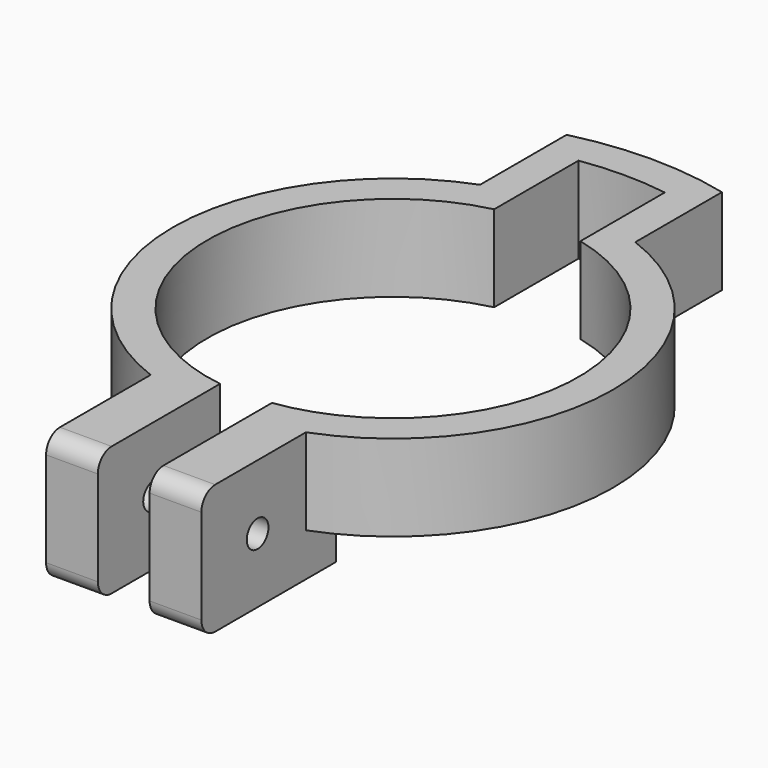
from build123d import *

# Parameters (mm, degrees)
F1_DEPTH = 5
F3_DEPTH = 7.5
F5_DEPTH = 7.5
F6_R     = 1
F7_R     = 0.7847872087
F8_DEPTH = 25


with BuildPart() as f1:
    # F0 (on Top) → F1 (new body)
    with BuildSketch(Plane.XY):
        with BuildLine():
            Line((-4.5, 18.2019916493), (-4.5, 11.9294802904))
            ThreePointArc((-4.5, 11.9294802904), (0, -12.75), (4.5, 11.9294802904))
            Line((4.5, 11.9294802904), (4.5, 18.2019916493))
            ThreePointArc((4.5, 18.2019916493), (0, 18.75), (-4.5, 18.2019916493))
        make_face()
        with BuildLine():
            ThreePointArc((2.5, 10.4552618332), (0, -10.75), (-2.5, 10.4552618332))
            Line((-2.5, 10.4552618332), (-2.5, 16.5623820751))
            ThreePointArc((-2.5, 16.5623820751), (0, 16.75), (2.5, 16.5623820751))
            Line((2.5, 16.5623820751), (2.5, 10.4552618332))
        make_face(mode=Mode.SUBTRACT)
    extrude(amount=F1_DEPTH)

    # F2 (on face) → F3 (join)
    with BuildSketch(Plane.XY.offset(5)):
        with BuildLine():
            ThreePointArc((4.5, -9.7628120949), (0, -10.75), (-4.5, -9.7628120949))
            Line((-4.5, -9.7628120949), (-4.5, -11.9294802904))
            ThreePointArc((-4.5, -11.9294802904), (0, -12.75), (4.5, -11.9294802904))
            Line((4.5, -11.9294802904), (4.5, -9.7628120949))
        make_face()
        with BuildLine():
            ThreePointArc((4.5, -11.9294802904), (0, -12.75), (-4.5, -11.9294802904))
            Line((-4.5, -11.9294802904), (-4.5, -19.5))
            Line((-4.5, -19.5), (4.5, -19.5))
            Line((4.5, -19.5), (4.5, -11.9294802904))
        make_face()
    extrude(amount=-F3_DEPTH)

    # F4 (on face) → F5 (cut, through all)
    with BuildSketch(Plane.XY.offset(5)):
        with BuildLine():
            ThreePointArc((1.5, -10.644834428), (0, -10.75), (-1.5, -10.644834428))
            Line((-1.5, -10.644834428), (-1.5, -19.5))
            Line((-1.5, -19.5), (1.5, -19.5))
            Line((1.5, -19.5), (1.5, -10.644834428))
        make_face()
    extrude(amount=-F5_DEPTH, mode=Mode.SUBTRACT)

    # F6
    f6_edges = [f1.edges().sort_by_distance(p)[0] for p in [
        (-3, -19.5, 5),
        (3, -19.5, 5),
        (3, -19.5, -2.5),
        (-3, -19.5, -2.5),
    ]]
    fillet(f6_edges, radius=F6_R)

    # F7 (on face) → F8 (cut)
    with BuildSketch(Plane(origin=(-4.5, 0, 0), x_dir=(0, -1, 0), z_dir=(-1, 0, 0))):
        with Locations((15.4294802904, 1.25)):
            Circle(F7_R)
    extrude(amount=-F8_DEPTH, mode=Mode.SUBTRACT)


solid = f1.part
